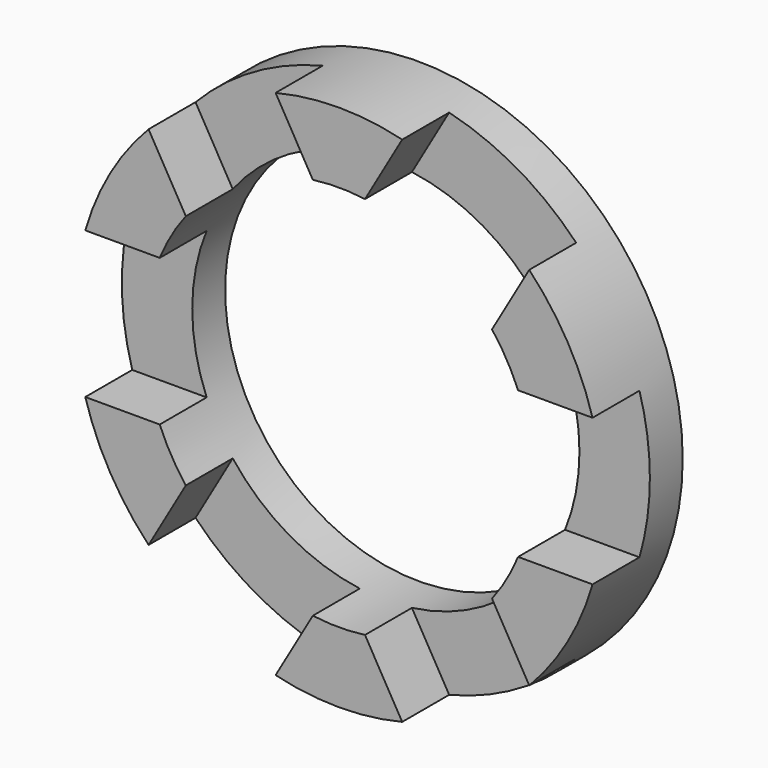
from build123d import *

# Parameters (mm, degrees)
F0_R            = 45
F0_R_2          = 33
F1_DEPTH        = 17
F2_R            = 5
F3_DEPTH        = 0.5
F3_COPIES_COUNT = 6
F6_DEPTH        = 10
F8_COUNT        = 6


# Not quite as in the source:
# - a pattern or mirror of a feature is missing from the dataset's text; its kind, count and spacing are read off the source's solid


with BuildPart() as f1:
    # F0 (on Front) → F1 (new body)
    with BuildSketch(Plane.XZ):
        Circle(F0_R)
        Circle(F0_R_2, mode=Mode.SUBTRACT)
    extrude(amount=F1_DEPTH)

    # F2 (on Front) → F3 (cut)
    with BuildSketch(Plane.XZ):
        with Locations((0, 39)):
            Circle(F2_R)
    f3 = extrude(amount=F3_DEPTH, mode=Mode.SUBTRACT)

    # F3_copies: F3 ×6 about axis
    f3_copies_axis = Axis((0, 0, 0), (0, 1, 0))
    for i in range(1, F3_COPIES_COUNT):
        add(f3.rotate(f3_copies_axis, i * 360 / F3_COPIES_COUNT), mode=Mode.SUBTRACT)

    # F5 (on face) → F6 (cut)
    with BuildSketch(Plane.XZ.offset(17)):
        with BuildLine():
            Line((-30.5409561082, 12.5), (-43.2290411645, 12.5))
            ThreePointArc((-43.2290411645, 12.5), (-45, 0), (-43.2290411645, -12.5))
            Line((-43.2290411645, -12.5), (-30.5409561082, -12.5))
            ThreePointArc((-30.5409561082, -12.5), (-33, 0), (-30.5409561082, 12.5))
        make_face()
    f6 = extrude(amount=-F6_DEPTH, mode=Mode.SUBTRACT)

    # F8: F6 ×6 about axis
    f8_axis = Axis((0, -20.116, 0), (0, -1, 0))
    for i in range(1, F8_COUNT):
        add(f6.rotate(f8_axis, i * 360 / F8_COUNT), mode=Mode.SUBTRACT)


solid = f1.part
